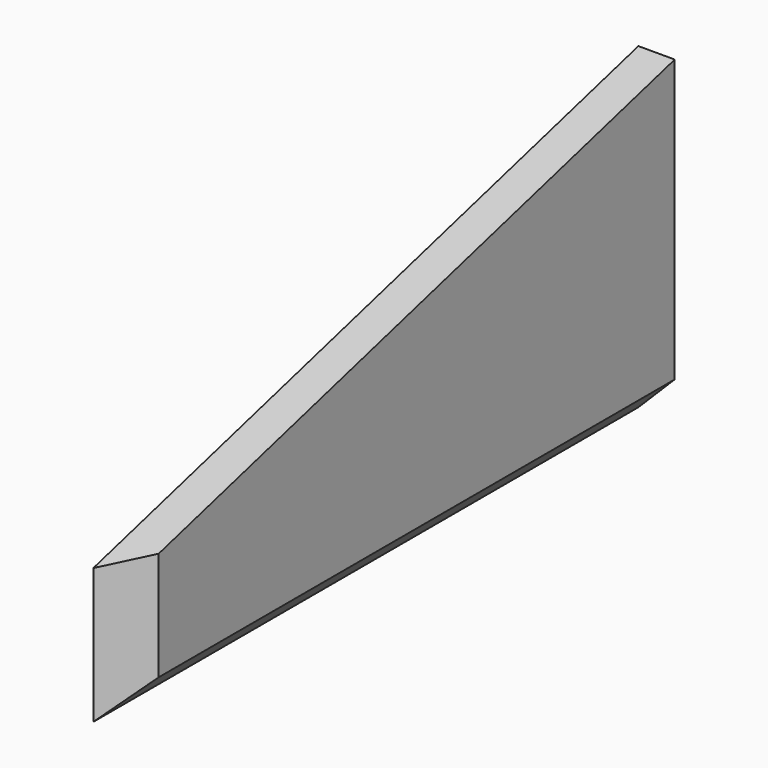
from build123d import *

# Parameters (mm, degrees)
F1_DEPTH = 16
F2_SIZE  = 15.99999


# Not quite as in the source:
# - a fillet or chamfer is up to 0.001 mm smaller than in the source, because OpenCascade refuses the exact size


with BuildPart() as f1:
    # F0 (on Right) → F1 (new body)
    with BuildSketch(Plane.YZ):
        Polygon((0, 59.6152422707), (0, 0), (300, 0), (300, 140), align=None)
    extrude(amount=F1_DEPTH)

    # F2 (size 16 in the source; OpenCascade refuses exactly that, so slightly less here)
    f2_edges = [f1.edges().sort_by_distance(p)[0] for p in [
        (16, 150, 0),
        (16, 0, 29.807621),
    ]]
    chamfer(f2_edges, length=F2_SIZE)


solid = f1.part
